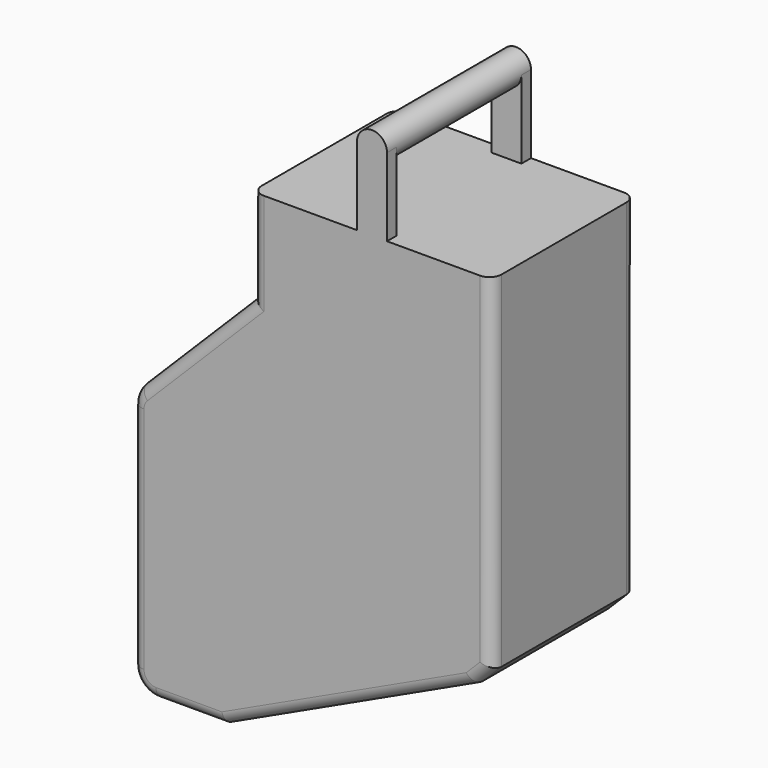
from build123d import *

# Parameters (mm, degrees)
F2_DEPTH  = 15
F3_R      = 2
F4_R      = 1
F7_DEPTH  = 15
F8_W      = 3.7031254775
F8_H      = 13
F9_DEPTH  = 25
F10_R     = 1.25
F11_DEPTH = 13


with BuildPart() as f2:
    # F1 (on Front) → F2 (new body)
    with BuildSketch(Plane.XZ):
        Polygon((10, 22.2655313462), (0, 12.2655313462), (0, -9.6663414017), (7.7085571088, -9.6663414017), (28.4380931407, 0), (30, 1.5619068593), (30, 30.3336585983), (10, 30.3336585983), align=None)
    extrude(amount=F2_DEPTH)

    # F3
    f3_edges = [f2.edges().sort_by_distance(p)[0] for p in [
        (0, -7.5, 12.265531),
        (0, -7.5, -9.666341),
    ]]
    fillet(f3_edges, radius=F3_R)

    # F4
    f4_edges = [f2.edges().sort_by_distance(p)[0] for p in [
        (5.292893, -15, 17.558425),
        (10, -15, 26.299595),
        (10, 0, 26.299595),
        (5.292893, 0, 17.558425),
        (18.073325, -15, -4.833171),
        (30, -15, 15.947783),
        (29.219047, -15, 0.780953),
        (29.219047, 0, 0.780953),
        (30, 0, 15.947783),
        (18.073325, 0, -4.833171),
        (0.152241, 0, 12.202471),
        (0, 0, 1.885381),
        (0.585786, 0, -9.080555),
        (4.854279, 0, -9.666341),
        (0.152241, -15, 12.202471),
        (0, -15, 1.885381),
        (0.585786, -15, -9.080555),
        (4.854279, -15, -9.666341),
    ]]
    fillet(f4_edges, radius=F4_R)

    # F6 (on Front) → F7 (join)
    with BuildSketch(Plane.XZ):
        with BuildLine():
            Line((18.75, 30.3336585983), (21.25, 30.3336585983))
            Line((21.25, 30.3336585983), (21.25, 36.8336585983))
            ThreePointArc((21.25, 36.8336585983), (20, 38.0836585983), (18.75, 36.8336585983))
            Line((18.75, 36.8336585983), (18.75, 30.3336585983))
        make_face()
    extrude(amount=F7_DEPTH)

    # F8 (on face) → F9 (cut)
    with BuildSketch(Plane.XY.offset(30.3336585983)):
        with Locations((20.149352029, -7.5)):
            Rectangle(F8_W, F8_H)
    extrude(amount=F9_DEPTH, mode=Mode.SUBTRACT)

    # F10 (on face) → F11 (join)
    with BuildSketch(Plane.XZ.offset(1)):
        with Locations((20, 36.8336585983)):
            Circle(F10_R)
    extrude(amount=F11_DEPTH)


solid = f2.part
